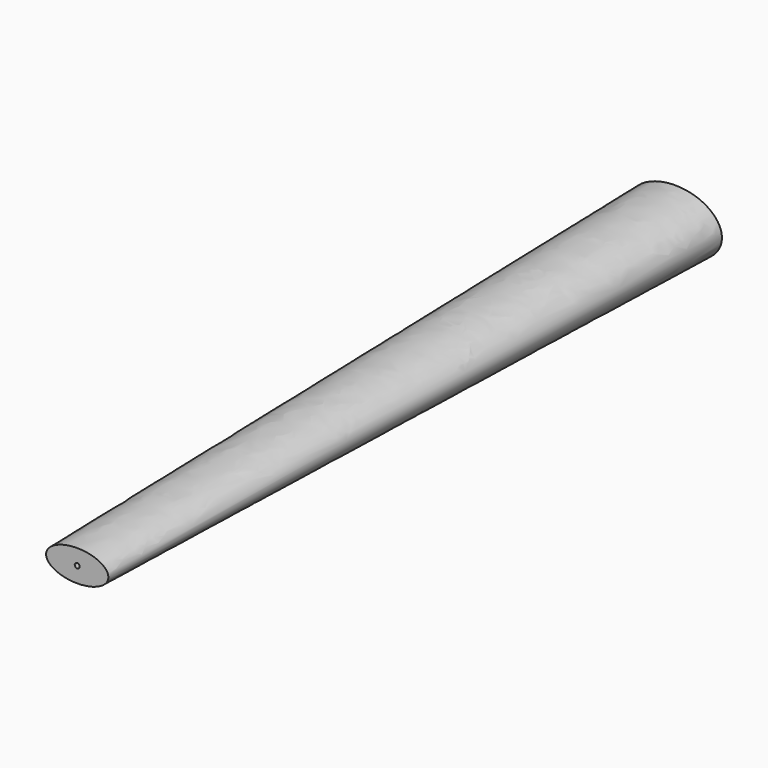
from build123d import *

# Parameters (mm, degrees)
F4_R     = 4
F5_DEPTH = 1200


with BuildPart() as f3:
    # F0 (on Front) → F3 section 0
    with BuildSketch(Plane.XZ):
        with BuildLine():
            add(Edge.make_bspline(
                [(75, 0), (75, 86.6025403784), (-37.5, 43.3012701892), (-150, 0), (-37.5, -43.3012701892), (75, -86.6025403784), (75, 0)],
                knots=[0, 0, 0, 2.0943951024, 2.0943951024, 4.1887902048, 4.1887902048, 6.2831853072, 6.2831853072, 6.2831853072], degree=2, weights=[1, 0.5, 1, 0.5, 1, 0.5, 1]))
        make_face()
    # F2 (on offset) → F3 section 1
    with BuildSketch(Plane.XZ.offset(1200)):
        with BuildLine():
            add(Edge.make_bspline(
                [(50, 0), (50, 43.3012701892), (-25, 21.6506350946), (-100, 0), (-25, -21.6506350946), (50, -43.3012701892), (50, 0)],
                knots=[0, 0, 0, 2.0943951024, 2.0943951024, 4.1887902048, 4.1887902048, 6.2831853072, 6.2831853072, 6.2831853072], degree=2, weights=[1, 0.5, 1, 0.5, 1, 0.5, 1]))
        make_face()
    loft()

    # F4 (on face) → F5 (cut)
    with BuildSketch(Plane(origin=(0, 0, 0), x_dir=(-1, 0, 0), z_dir=(0, 1, 0))):
        Circle(F4_R)
    extrude(amount=-F5_DEPTH, mode=Mode.SUBTRACT)


solid = f3.part
